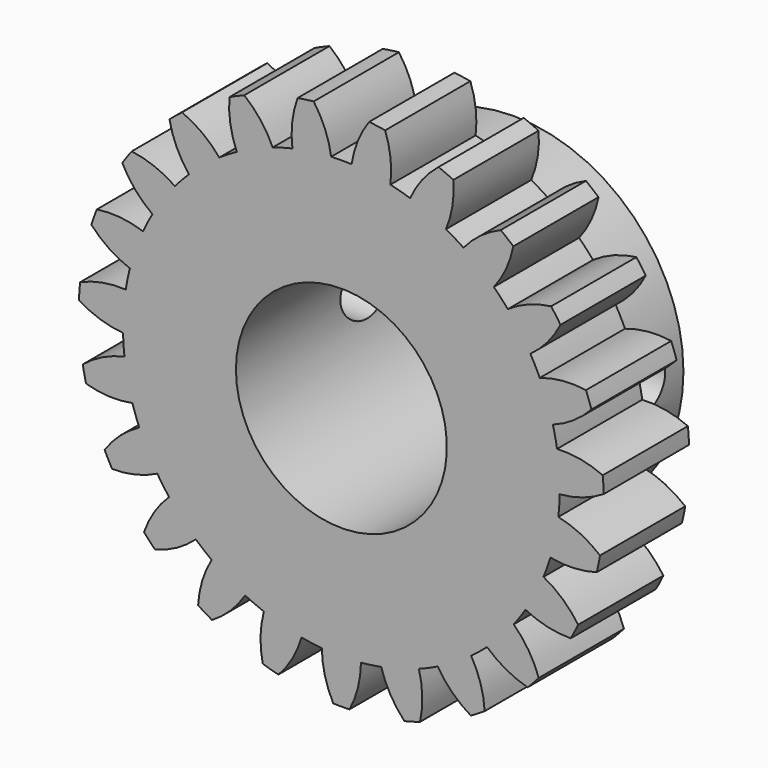
from build123d import *

# Parameters (mm, degrees)
F2_R            = 9.9
F3_DEPTH        = 25
F5_DEPTH        = 25
F5_COPIES_COUNT = 23
F7_R            = 2.95
F8_DEPTH        = 37.3


# Not quite as in the source:
# - a feature of the source that left no trace in its solid (it failed there, or was rolled back) is left out
# - a pattern or mirror of a feature is missing from the dataset's text; its kind, count and spacing are read off the source's solid


with BuildPart() as f1:
    # F0 (on Right) → F1 (revolve)
    with BuildSketch(Plane.YZ):
        Polygon((0, 24.65), (0, 0), (20.2, 0), (20.2, 15.95), (10, 15.95), (10, 24.65), align=None)
    revolve(axis=Axis((0, 10.1, 0), (0, 1, 0)))

    # F2 (on face) → F3 (cut)
    with BuildSketch(Plane(origin=(0, 20.2, 0), x_dir=(-1, 0, 0), z_dir=(0, 1, 0))):
        Circle(F2_R)
    extrude(amount=-F3_DEPTH, mode=Mode.SUBTRACT)

    # F4 (on face) → F5 (cut)
    with BuildSketch(Plane.XZ):
        with BuildLine():
            ThreePointArc((0.9605272399, 20.4764837905), (1.5385061373, 22.5929437067), (2.6011700561, 24.5123726787))
            ThreePointArc((2.6011700561, 24.5123726787), (0, 24.65), (-2.6011700561, 24.5123726787))
            ThreePointArc((-2.6011700561, 24.5123726787), (-1.5385061373, 22.5929437067), (-0.9605272399, 20.4764837905))
            ThreePointArc((-0.9605272399, 20.4764837905), (0, 20.499), (0.9605272399, 20.4764837905))
        make_face()
        with BuildLine():
            ThreePointArc((2.6011700561, 24.5123726787), (2.8144449637, 24.7961797548), (3.0385106282, 25.0715471833))
            ThreePointArc((3.0385106282, 25.0715471833), (0, 25.255), (-3.0385106282, 25.0715471833))
            ThreePointArc((-3.0385106282, 25.0715471833), (-2.8144449637, 24.7961797548), (-2.6011700561, 24.5123726787))
            ThreePointArc((-2.6011700561, 24.5123726787), (0, 24.65), (2.6011700561, 24.5123726787))
        make_face()
    f5 = extrude(amount=-F5_DEPTH, mode=Mode.SUBTRACT)

    # F5_copies: F5 ×23 about axis
    f5_copies_axis = Axis((0, 0, 0), (0, 1, 0))
    for i in range(1, F5_COPIES_COUNT):
        add(f5.rotate(f5_copies_axis, i * 360 / F5_COPIES_COUNT), mode=Mode.SUBTRACT)

    # F7 (on Right) → F8 (cut, symmetric)
    with BuildSketch(Plane.YZ):
        with Locations((15.15, 1.0436970042)):
            Circle(F7_R)
    extrude(amount=F8_DEPTH, both=True, mode=Mode.SUBTRACT)


solid = f1.part
